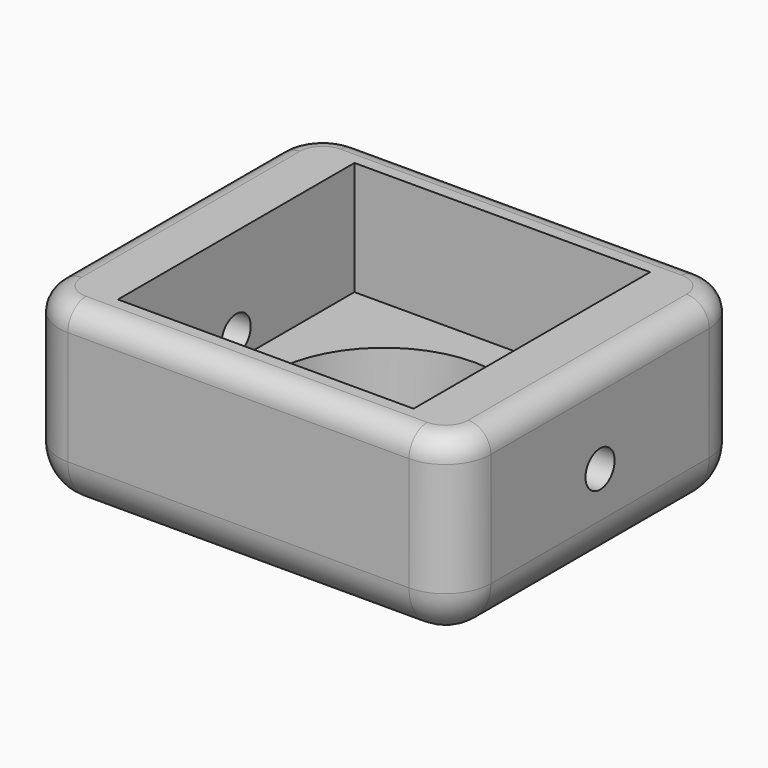
from build123d import *

# Parameters (mm, degrees)
F0_W         = 19
F0_H         = 16
F0_W_2       = 13
F0_H_2       = 13
F0_R         = 5
F1_DEPTH     = 3
F2_W         = 19
F2_H         = 16
F2_W_2       = 13
F2_H_2       = 13
F3_DEPTH     = 5
F5_D         = 1.6
F6_R         = 2
F7_T1_DEPTH  = 11
F7_S5_W      = 2
F7_S5_H      = 2
F7_T6_DEPTH  = 2
F7_S11_W     = 2
F7_S11_H     = 2
F7_T12_DEPTH = 2
F7_S17_W     = 2
F7_S17_H     = 2
F7_T18_DEPTH = 2
F7_S23_W     = 2
F7_S23_H     = 2
F7_T24_DEPTH = 2
F8_R         = 1


# Not quite as in the source:
# - a fillet or chamfer that OpenCascade refuses, or shapes differently, is made with other operations: its cross-section is extruded or revolved along the edge and cut away or added


with BuildPart() as f1:
    # F0 (on Top) → F1 (new body)
    with BuildSketch(Plane.XY):
        Rectangle(F0_W, F0_H)
        Rectangle(F0_W_2, F0_H_2, mode=Mode.SUBTRACT)
        Rectangle(F0_W_2, F0_H_2)
        Circle(F0_R, mode=Mode.SUBTRACT)
    extrude(amount=F1_DEPTH)

    # F2 (on face) → F3 (join)
    with BuildSketch(Plane.XY.offset(3)):
        Rectangle(F2_W, F2_H)
        Rectangle(F2_W_2, F2_H_2, mode=Mode.SUBTRACT)
    extrude(amount=F3_DEPTH)

    # F5 (through all)
    with Locations(Plane.YZ.offset(9.5)):
        with Locations((0, 4)):
            Hole(F5_D / 2)

    # F6
    f6_edges = [f1.edges().sort_by_distance(p)[0] for p in [
        (0, -8, 0),
        (0, 8, 0),
        (-9.5, 0, 0),
        (9.5, 0, 0),
    ]]
    fillet(f6_edges, radius=F6_R)

    # F7: fillet of radius 2 on 4 edges, made by hand

    # F7_s2 → F7_t1 (cut)
    with BuildSketch(Plane.XY.offset(2)):
        with BuildLine():
            ThreePointArc((9.5, -6), (8.9142135624, -7.4142135624), (7.5, -8))
            Line((7.5, -8), (9.5, -8))
            Line((9.5, -8), (9.5, -6))
        make_face()
        with BuildLine():
            ThreePointArc((9.5, 6), (8.9142135624, 7.4142135624), (7.5, 8))
            Line((7.5, 8), (9.5, 8))
            Line((9.5, 8), (9.5, 6))
        make_face()
        with BuildLine():
            ThreePointArc((-7.5, -8), (-8.9142135624, -7.4142135624), (-9.5, -6))
            Line((-9.5, -6), (-9.5, -8))
            Line((-9.5, -8), (-7.5, -8))
        make_face()
        with BuildLine():
            ThreePointArc((-7.5, 8), (-8.9142135624, 7.4142135624), (-9.5, 6))
            Line((-9.5, 6), (-9.5, 8))
            Line((-9.5, 8), (-7.5, 8))
        make_face()
    extrude(amount=F7_T1_DEPTH, mode=Mode.SUBTRACT)


with BuildPart() as f7_tool4:
    # F7_s5 → F7_t6 (new body)
    with BuildSketch(Plane.XZ.offset(-6)):
        with Locations((-8.5, 1)):
            Rectangle(F7_S5_W, F7_S5_H)
    extrude(amount=-F7_T6_DEPTH)

    # F7_s7 → F7_t8 (revolve, cut)
    with BuildSketch(Plane(origin=(-7.5, 6, 2), x_dir=(0.7071067812, 0, 0.7071067812), z_dir=(-0.7071067812, 0, 0.7071067812))):
        with BuildLine():
            ThreePointArc((0, -2), (2, 0), (0, 2))
            Line((0, 2), (0, -2))
        make_face()
    revolve(axis=Axis((-7.5, 6, 2), (0, 1, 0)), mode=Mode.SUBTRACT)


with BuildPart() as f1_1:
    add(f1.part)

    # F7_t3: cut F7_tool4
    add(f7_tool4.part, mode=Mode.SUBTRACT)


with BuildPart() as f7_tool10:
    # F7_s11 → F7_t12 (new body)
    with BuildSketch(Plane.XZ.offset(6)):
        with Locations((-8.5, 1)):
            Rectangle(F7_S11_W, F7_S11_H)
    extrude(amount=F7_T12_DEPTH)

    # F7_s13 → F7_t14 (revolve, cut)
    with BuildSketch(Plane(origin=(-7.5, -6, 2), x_dir=(0.7071067812, 0, 0.7071067812), z_dir=(0.7071067812, 0, -0.7071067812))):
        with BuildLine():
            ThreePointArc((0, -2), (2, 0), (0, 2))
            Line((0, 2), (0, -2))
        make_face()
    revolve(axis=Axis((-7.5, -6, 2), (0, -1, 0)), mode=Mode.SUBTRACT)


with BuildPart() as f1_2:
    add(f1_1.part)

    # F7_t9: cut F7_tool10
    add(f7_tool10.part, mode=Mode.SUBTRACT)


with BuildPart() as f7_tool16:
    # F7_s17 → F7_t18 (new body)
    with BuildSketch(Plane.YZ.offset(7.5)):
        with Locations((7, 1)):
            Rectangle(F7_S17_W, F7_S17_H)
    extrude(amount=F7_T18_DEPTH)

    # F7_s19 → F7_t20 (revolve, cut)
    with BuildSketch(Plane(origin=(7.5, 6, 2), x_dir=(0, -0.7071067812, 0.7071067812), z_dir=(0, 0.7071067812, 0.7071067812))):
        with BuildLine():
            ThreePointArc((0, -2), (2, 0), (0, 2))
            Line((0, 2), (0, -2))
        make_face()
    revolve(axis=Axis((7.5, 6, 2), (1, 0, 0)), mode=Mode.SUBTRACT)


with BuildPart() as f1_3:
    add(f1_2.part)

    # F7_t15: cut F7_tool16
    add(f7_tool16.part, mode=Mode.SUBTRACT)


with BuildPart() as f7_tool22:
    # F7_s23 → F7_t24 (new body)
    with BuildSketch(Plane.YZ.offset(7.5)):
        with Locations((-7, 1)):
            Rectangle(F7_S23_W, F7_S23_H)
    extrude(amount=F7_T24_DEPTH)

    # F7_s25 → F7_t26 (revolve, cut)
    with BuildSketch(Plane(origin=(7.5, -6, 2), x_dir=(0, 0.7071067812, 0.7071067812), z_dir=(0, 0.7071067812, -0.7071067812))):
        with BuildLine():
            ThreePointArc((0, -2), (2, 0), (0, 2))
            Line((0, 2), (0, -2))
        make_face()
    revolve(axis=Axis((7.5, -6, 2), (1, 0, 0)), mode=Mode.SUBTRACT)


with BuildPart() as f1_4:
    add(f1_3.part)

    # F7_t21: cut F7_tool22
    add(f7_tool22.part, mode=Mode.SUBTRACT)

    # F8
    f8_edges = [f1_4.edges().sort_by_distance(p)[0] for p in [
        (0, 8, 8),
    ]]
    fillet(f8_edges, radius=F8_R)


solid = f1_4.part
